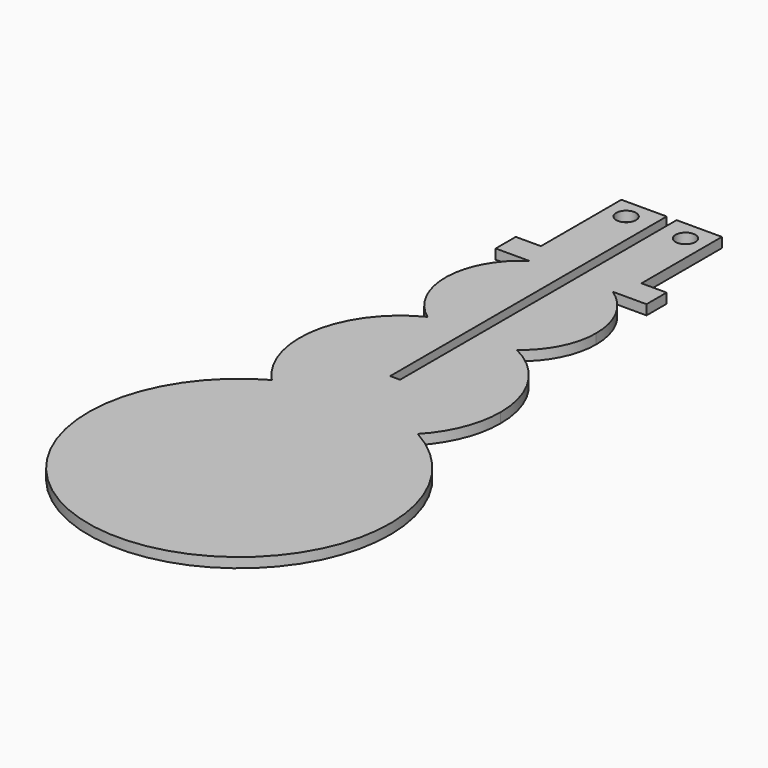
from build123d import *

# Parameters (mm, degrees)
F0_W     = 11.45
F0_H     = 25.4
F0_R     = 2.5
F1_DEPTH = 2.5


# Not quite as in the source:
# - a feature names something its author has since deleted; it is built from what else it names


with BuildPart() as f1:
    # F0 (on Top) → F1 (new body)
    with BuildSketch(Plane.XY):
        with Locations((6.975, 73.025)):
            Rectangle(F0_W, F0_H)
        with Locations((7.5, 80.725)):
            Circle(F0_R, mode=Mode.SUBTRACT)
        with Locations((-6.975, 73.025)):
            Rectangle(F0_W, F0_H)
        with Locations((-7.5, 80.725)):
            Circle(F0_R, mode=Mode.SUBTRACT)
        with BuildLine():
            ThreePointArc((-10.5302837094, 53.975), (-6.0950122474, 56.1486377797), (-1.25, 57.1089452627))
            Line((-1.25, 57.1089452627), (-1.25, 60.325))
            Line((-1.25, 60.325), (-12.7, 60.325))
            Line((-12.7, 60.325), (-19.05, 60.325))
            Line((-19.05, 60.325), (-19.05, 53.975))
            Line((-19.05, 53.975), (-10.5302837094, 53.975))
        make_face()
        with BuildLine():
            ThreePointArc((1.25, 57.1089452627), (6.0950122474, 56.1486377797), (10.5302837094, 53.975))
            Line((10.5302837094, 53.975), (19.05, 53.975))
            Line((19.05, 53.975), (19.05, 60.325))
            Line((19.05, 60.325), (12.7, 60.325))
            Line((12.7, 60.325), (1.25, 60.325))
            Line((1.25, 60.325), (1.25, 57.1089452627))
        make_face()
        with BuildLine():
            Line((1.25, 53.975), (10.5302837094, 53.975))
            ThreePointArc((10.5302837094, 53.975), (6.0950122474, 56.1486377797), (1.25, 57.1089452627))
            Line((1.25, 57.1089452627), (1.25, 53.975))
        make_face()
        with BuildLine():
            Line((-1.25, 53.975), (-1.25, 57.1089452627))
            ThreePointArc((-1.25, 57.1089452627), (-6.0950122474, 56.1486377797), (-10.5302837094, 53.975))
            Line((-10.5302837094, 53.975), (-1.25, 53.975))
        make_face()
        with BuildLine():
            Line((-1.25, 25.3692234804), (-1.25, 53.975))
            Line((-1.25, 53.975), (-10.5302837094, 53.975))
            ThreePointArc((-10.5302837094, 53.975), (-19.0443993724, 38.5619010114), (-11.2875107666, 22.7541666667))
            ThreePointArc((-11.2875107666, 22.7541666667), (-6.4036649343, 24.5795255326), (-1.25, 25.3692234804))
        make_face()
        with BuildLine():
            ThreePointArc((11.2875107666, 22.7541666667), (16.9989643817, 29.5012960309), (19.05, 38.1))
            ThreePointArc((19.05, 38.1), (16.785475934, 47.1083460007), (10.5302837094, 53.975))
            Line((10.5302837094, 53.975), (1.25, 53.975))
            Line((1.25, 53.975), (1.25, 25.3692234804))
            ThreePointArc((1.25, 25.3692234804), (6.4036649343, 24.5795255326), (11.2875107666, 22.7541666667))
        make_face()
        with BuildLine():
            ThreePointArc((-11.2875107666, 22.7541666667), (-6.5308415466, 20.204452825), (-1.25, 19.0910547373))
            Line((-1.25, 19.0910547373), (-1.25, 25.3692234804))
            ThreePointArc((-1.25, 25.3692234804), (-6.4036649343, 24.5795255326), (-11.2875107666, 22.7541666667))
        make_face()
        with BuildLine():
            ThreePointArc((1.25, 19.0910547373), (6.5308415466, 20.204452825), (11.2875107666, 22.7541666667))
            ThreePointArc((11.2875107666, 22.7541666667), (6.4036649343, 24.5795255326), (1.25, 25.3692234804))
            Line((1.25, 25.3692234804), (1.25, 19.0910547373))
        make_face()
        with BuildLine():
            ThreePointArc((-18.4450831863, -17.4625), (0, -25.4), (18.4450831863, -17.4625))
            ThreePointArc((18.4450831863, -17.4625), (0, -12.7), (-18.4450831863, -17.4625))
        make_face()
        with BuildLine():
            ThreePointArc((38.1, -50.8), (32.820478892, -31.4499052896), (18.4450831863, -17.4625))
            ThreePointArc((18.4450831863, -17.4625), (0, -25.4), (-18.4450831863, -17.4625))
            ThreePointArc((-18.4450831863, -17.4625), (-19.3500947104, -83.620478892), (38.1, -50.8))
        make_face()
        with BuildLine():
            ThreePointArc((25.4, 0), (21.5854438624, 13.3876291129), (11.2875107666, 22.7541666667))
            ThreePointArc((11.2875107666, 22.7541666667), (6.5308415466, 20.204452825), (1.25, 19.0910547373))
            Line((1.25, 19.0910547373), (1.25, -1.5875))
            Line((1.25, -1.5875), (-1.25, -1.5875))
            Line((-1.25, -1.5875), (-1.25, 19.0910547373))
            ThreePointArc((-1.25, 19.0910547373), (-6.5308415466, 20.204452825), (-11.2875107666, 22.7541666667))
            ThreePointArc((-11.2875107666, 22.7541666667), (-25.0070361146, 4.4506341979), (-18.4450831863, -17.4625))
            ThreePointArc((-18.4450831863, -17.4625), (0, -12.7), (18.4450831863, -17.4625))
            ThreePointArc((18.4450831863, -17.4625), (23.5972997707, -9.3982681135), (25.4, 0))
        make_face()
    extrude(amount=F1_DEPTH)


solid = f1.part
